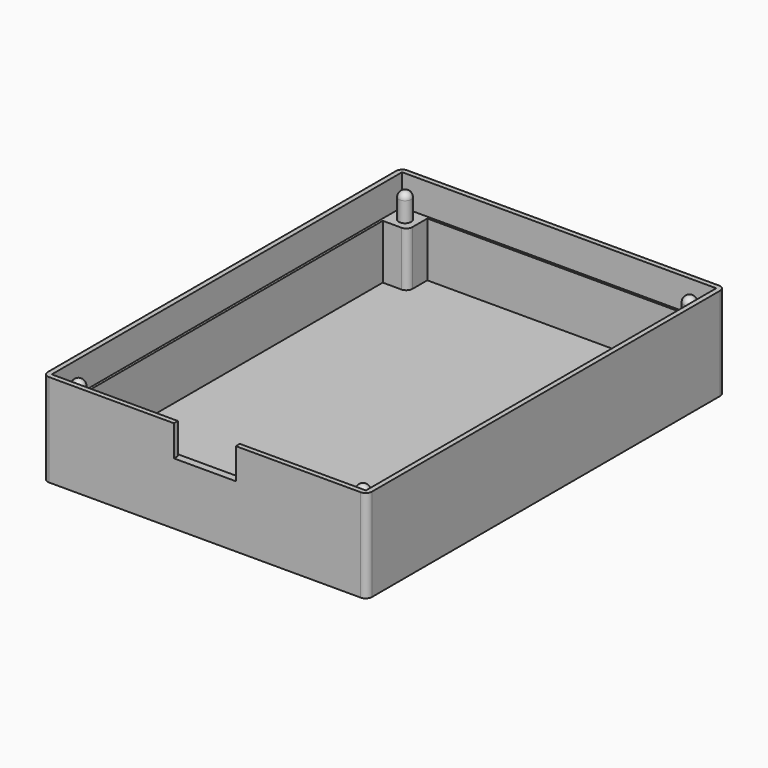
from build123d import *

# Parameters (mm, degrees)
F1_W      = 52.4
F1_H      = 72.4
F2_DEPTH  = 15
F3_T      = -1.2
F0_R      = 1
F4_DEPTH  = 10
F5_DEPTH  = 13
F6_R      = 1
F8_W      = 50.8
F8_H      = 70.8
F8_W_2    = 50
F8_H_2    = 70
F9_DEPTH  = 5
F10_W     = 10
F10_H     = 10
F11_DEPTH = 25


# Not quite as in the source:
# - two fillets or chamfers of one size are made in one step


with BuildPart() as f2:
    # F1 (on Top) → F2 (new body)
    with BuildSketch(Plane.XY):
        with Locations((25, 35)):
            Rectangle(F1_W, F1_H)
    extrude(amount=F2_DEPTH)

    # F3
    f3_openings = [f2.faces().sort_by_distance(p)[0] for p in [
        (25, 35, 15),
    ]]
    offset(amount=F3_T, openings=f3_openings)

    # F0 (on Top) → F4 (join)
    with BuildSketch(Plane.XY):
        with BuildLine():
            Line((4, 70), (0, 70))
            Line((0, 70), (0, 66))
            Line((0, 66), (3, 66))
            ThreePointArc((3, 66), (3.7071067812, 66.2928932188), (4, 67))
            Line((4, 67), (4, 70))
        make_face()
        with Locations((2, 68)):
            Circle(F0_R, mode=Mode.SUBTRACT)
        with BuildLine():
            Line((47, 66), (50, 66))
            Line((50, 66), (50, 70))
            Line((50, 70), (46, 70))
            Line((46, 70), (46, 67))
            ThreePointArc((46, 67), (46.2928932188, 66.2928932188), (47, 66))
        make_face()
        with Locations((48, 68)):
            Circle(F0_R, mode=Mode.SUBTRACT)
        with BuildLine():
            Line((50, 0), (50, 4))
            Line((50, 4), (47, 4))
            ThreePointArc((47, 4), (46.2928932188, 3.7071067812), (46, 3))
            Line((46, 3), (46, 0))
            Line((46, 0), (50, 0))
        make_face()
        with Locations((48, 2)):
            Circle(F0_R, mode=Mode.SUBTRACT)
        with BuildLine():
            ThreePointArc((4, 3), (3.7071067812, 3.7071067812), (3, 4))
            Line((3, 4), (0, 4))
            Line((0, 4), (0, 0))
            Line((0, 0), (4, 0))
            Line((4, 0), (4, 3))
        make_face()
        with Locations((2, 2)):
            Circle(F0_R, mode=Mode.SUBTRACT)
    extrude(amount=F4_DEPTH)

    # F5 (add): faces of the model
    f5_faces = [f2.faces().sort_by_distance(p)[0] for p in [
        (2, 2, 1.2),
        (48, 2, 1.2),
        (2, 68, 1.2),
        (48, 68, 1.2),
    ]]
    extrude(f5_faces, amount=F5_DEPTH)

    # F6
    f6_edges = [f2.edges().sort_by_distance(p)[0] for p in [
        (1, 2, 14.2),
        (47, 2, 14.2),
        (1, 68, 14.2),
        (47, 68, 14.2),
        (-1.2, -1.2, 7.5),
        (51.2, -1.2, 7.5),
        (-1.2, 71.2, 7.5),
        (51.2, 71.2, 7.5),
    ]]
    fillet(f6_edges, radius=F6_R)

    # F8 (on face) → F9 (cut)
    with BuildSketch(Plane.XY.offset(15)):
        with Locations((25, 35)):
            Rectangle(F8_W, F8_H)
        with Locations((25, 35)):
            Rectangle(F8_W_2, F8_H_2, mode=Mode.SUBTRACT)
    extrude(amount=-F9_DEPTH, mode=Mode.SUBTRACT)

    # F10 (on face) → F11 (cut)
    with BuildSketch(Plane.XZ.offset(1.2)):
        with Locations((25, 15)):
            Rectangle(F10_W, F10_H)
    extrude(amount=-F11_DEPTH, mode=Mode.SUBTRACT)


solid = f2.part
